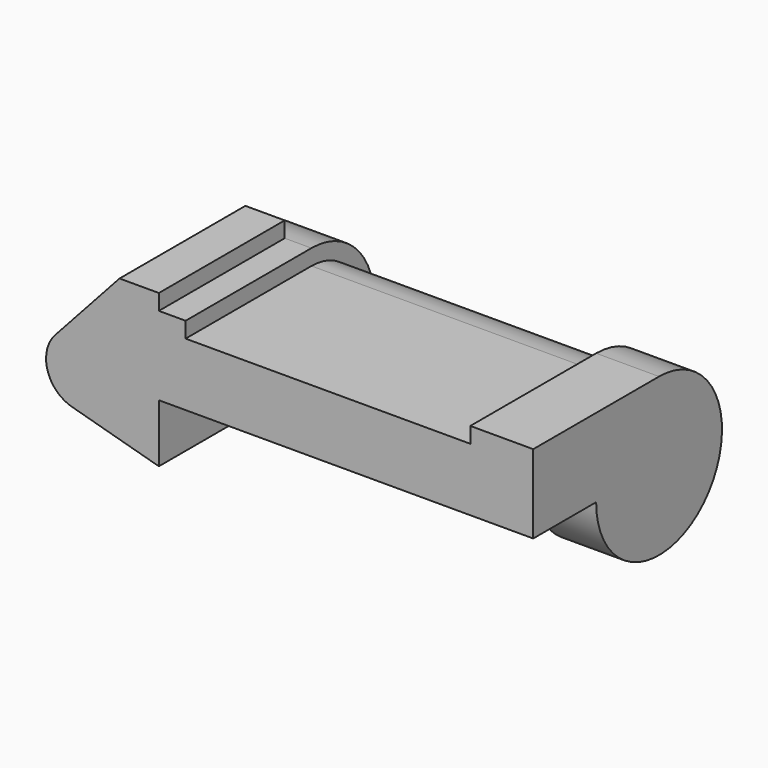
from build123d import *

# Parameters (mm, degrees)
F0_W     = 5.842
F0_H     = 12.7
F0_R     = 3.175
F2_DEPTH = 25.4


with BuildPart() as f1:
    # F0 (on Front) → F1 (revolve)
    with BuildSketch(Plane.XZ):
        Polygon((5.842, 12.7), (5.842, 0), (66.294, 0), (66.294, 12.7), (56.134, 12.7), (56.134, 10.16), (10.16, 10.16), (10.16, 12.7), align=None)
        with Locations((2.921, 6.35)):
            Rectangle(F0_W, F0_H)
    revolve(axis=Axis((33.147, 0, 0), (-1, 0, 0)))

    # F0 (on Front) → F2 (join)
    with BuildSketch(Plane.XZ):
        Polygon((5.842, 12.7), (5.842, 0), (66.294, 0), (66.294, 12.7), (56.134, 12.7), (56.134, 10.16), (10.16, 10.16), (10.16, 12.7), align=None)
        with BuildLine():
            ThreePointArc((-8.1826630726, -5.5069827884), (-3.1957909266, -4.5493385486), (-0.9398, 0))
            ThreePointArc((-0.9398, 0), (-4.5919612295, 5.3297205562), (-10.8806298187, 3.8475430269))
            ThreePointArc((-10.8806298187, 3.8475430269), (-12.1459778134, -1.5837270034), (-8.1826630726, -5.5069827884))
        make_face()
        with Locations((-6.6548, 0)):
            Circle(F0_R, mode=Mode.SUBTRACT)
        with BuildLine():
            Line((-0.9398, 0), (0, 0))
            Line((0, 0), (0, 12.7))
            Line((0, 12.7), (5.842, 12.7))
            Line((5.842, 12.7), (5.842, 15.24))
            Line((5.842, 15.24), (-0.508, 15.24))
            Line((-0.508, 15.24), (-10.8806298187, 3.8475430269))
            ThreePointArc((-10.8806298187, 3.8475430269), (-4.5919612295, 5.3297205562), (-0.9398, 0))
        make_face()
        with Locations((2.921, 6.35)):
            Rectangle(F0_W, F0_H)
        with BuildLine():
            Line((5.842, 0), (0, 0))
            Line((0, 0), (-0.9398, 0))
            ThreePointArc((-0.9398, 0), (-3.1957909266, -4.5493385486), (-8.1826630726, -5.5069827884))
            Line((-8.1826630726, -5.5069827884), (5.842, -9.398))
            Line((5.842, -9.398), (5.842, 0))
        make_face()
        with Locations((-6.6548, 0)):
            Circle(F0_R)
    extrude(amount=F2_DEPTH)


solid = f1.part
